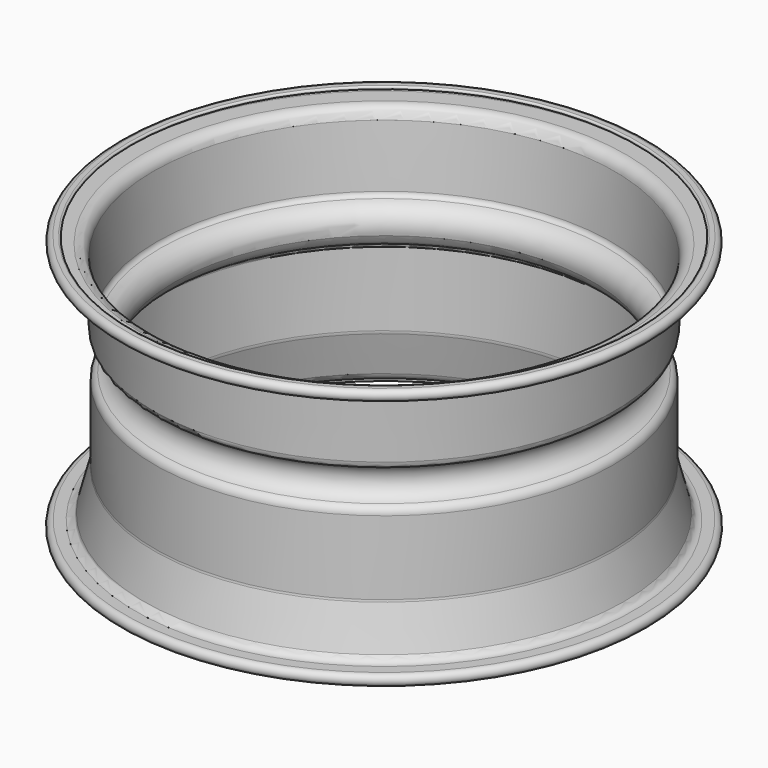
from build123d import *


# Not quite as in the source:
# - ends of sketch curves that miss each other by under 0.0002 mm in the source are joined


with BuildPart() as f1:
    # F0 (on Front) → F1 (revolve)
    with BuildSketch(Plane.XZ):
        with BuildLine():
            Line((-119.8179203278, -19.0465514287), (-125.9695880596, -19.0465514287))
            ThreePointArc((-125.9695880596, -19.0465514287), (-129.3662774079, -22.443240777), (-125.9695880596, -25.8399301254))
            Line((-125.9695880596, -25.8399301254), (-124.844422109, -25.8399301254))
            ThreePointArc((-124.844422109, -25.8399301254), (-123.844422109, -24.8399301254), (-124.844422109, -23.8399301254))
            Line((-124.844422109, -23.8399301254), (-126.1090040207, -23.8399301254))
            ThreePointArc((-126.1090040207, -23.8399301254), (-127.505693369, -22.443240777), (-126.1090040207, -21.0465514287))
            Line((-126.1090040207, -21.0465514287), (-119.8179203278, -21.0465514287))
            ThreePointArc((-119.8179203278, -21.0465514287), (-115.5484267824, -19.5937511607), (-113.051139342, -15.8383871048))
            Line((-113.051139342, -15.8383871048), (-106.5235113191, 8.8128852061))
            ThreePointArc((-106.5235113191, 8.8128852061), (-106.3488419197, 9.7012461733), (-106.2902923049, 10.6047208822))
            Line((-106.2902923049, 10.6047208822), (-106.2902923049, 55.3422208118))
            ThreePointArc((-106.2902923049, 55.3422208118), (-105.7338143755, 57.0879527893), (-104.265837153, 58.1844429614))
            ThreePointArc((-104.265837153, 58.1844429614), (-99.325868004, 61.3552385973), (-96.4025768764, 66.445583295))
            ThreePointArc((-96.4025768764, 66.445583295), (-97.4669768084, 75.8898468365), (-104.9141860429, 81.7946021806))
            ThreePointArc((-104.9141860429, 81.7946021806), (-106.4411114383, 82.8101122267), (-107.0917370222, 84.5245941211))
            Line((-107.0917370222, 84.5245941211), (-109.1232600955, 121.4868285056))
            ThreePointArc((-109.1232600955, 121.4868285056), (-109.1237491724, 121.4952214879), (-109.1241919641, 121.5036170425))
            ThreePointArc((-109.1241919641, 121.5036170425), (-111.2986521131, 126.2117189643), (-116.1158979645, 128.1323030038))
            Line((-116.1158979645, 128.1323030038), (-126.2164527022, 128.1323030038))
            ThreePointArc((-126.2164527022, 128.1323030038), (-127.4648065061, 129.3806568078), (-126.2164527022, 130.6290106117))
            Line((-126.2164527022, 130.6290106117), (-123.416104953, 130.6290106117))
            ThreePointArc((-123.416104953, 130.6290106117), (-122.416104953, 131.6290106117), (-123.416104953, 132.6290106117))
            Line((-123.416104953, 132.6290106117), (-126.1158402698, 132.6290106117))
            ThreePointArc((-126.1158402698, 132.6290106117), (-129.2187648573, 129.3091583717), (-125.9695880596, 126.1323030038))
            Line((-125.9695880596, 126.1323030038), (-116.1158979645, 126.1323030038))
            ThreePointArc((-116.1158979645, 126.1323030038), (-112.6776149261, 124.7631043258), (-111.1217890692, 121.4051434602))
            Line((-111.1217890692, 121.4051434602), (-109.0890375897, 84.4205590276))
            ThreePointArc((-109.0890375897, 84.4205590276), (-108.0005653329, 81.5710411847), (-105.4591013497, 79.8841847552))
            ThreePointArc((-105.4591013497, 79.8841847552), (-97.9047348476, 70.1731016366), (-104.9147794404, 60.0620748147))
            ThreePointArc((-104.9147794404, 60.0620748147), (-107.3598399258, 58.2382867202), (-108.2902923049, 55.3333285171))
            Line((-108.2902923049, 55.3333285171), (-108.2902923049, 10.6047208822))
            ThreePointArc((-108.2902923049, 10.6047208822), (-108.3321134583, 9.9593818044), (-108.456877315, 9.3248382564))
            Line((-108.456877315, 9.3248382564), (-114.9845053379, -15.3264340545))
            ThreePointArc((-114.9845053379, -15.3264340545), (-116.7682820811, -18.0088369515), (-119.8179203278, -19.0465514287))
        make_face()
    revolve(axis=Axis((30.6312496229, 0, 51.8589288074), (0, 0, -1)))


solid = f1.part
